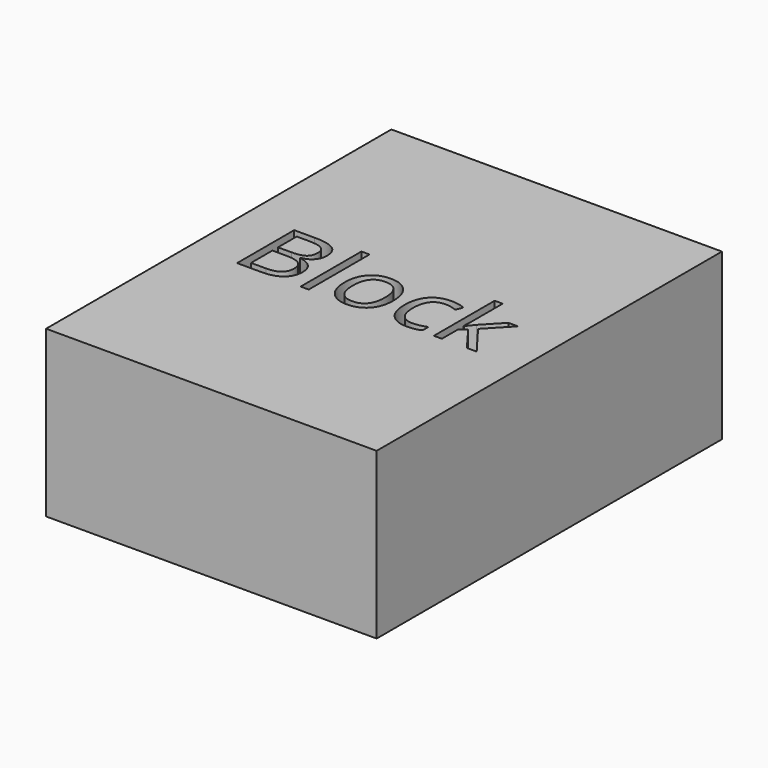
from build123d import *

# Parameters (mm, degrees)
F0_W         = 91.44
F0_H         = 119.38
F1_DEPTH     = 45.72
F2_TEXT_SIZE = 27.6484909182
F3_DEPTH     = 6.35


# Not quite as in the source:
# - Text() gives the source's letters only with a copy of the font that has no kerning and outlines rounded to 1/6400 em; it was checked with that copy


with BuildPart() as f1:
    # F0 (on Top) → F1 (new body)
    with BuildSketch(Plane.XY):
        with Locations((45.72, 59.69)):
            Rectangle(F0_W, F0_H)
    extrude(amount=F1_DEPTH)

    # F2 (on face) → F3 (cut)
    with BuildSketch(Plane.XY.offset(45.72)):
        with Locations((10.3277715863, 49.7365432694)):
            Text('Block', F2_TEXT_SIZE, font='Open Sans', text_align=(TextAlign.LEFT, TextAlign.BOTTOM))
    extrude(amount=-F3_DEPTH, mode=Mode.SUBTRACT)


solid = f1.part
